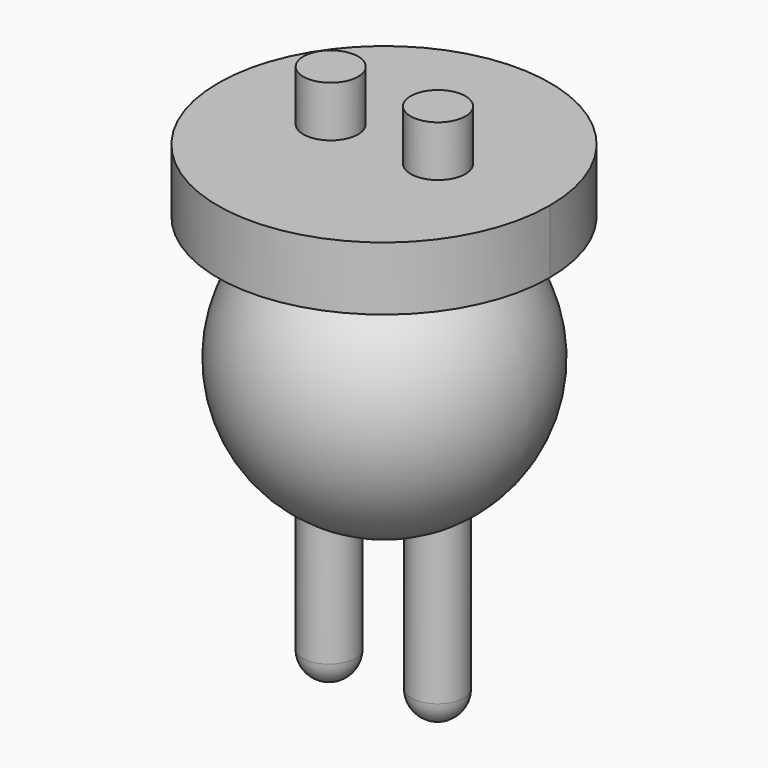
from build123d import *

# Parameters (mm, degrees)
F0_R     = 10.7853529021
F7_DEPTH = 45
F0_R_2   = 65.2735484533
F8_DEPTH = 25


with BuildPart() as f2:
    # F1 (on Front) → F2 (revolve)
    with BuildSketch(Plane.XZ):
        with BuildLine():
            ThreePointArc((0, -105.0551608205), (39.6174808002, -88.645062966), (56.0275786547, -49.0275821658))
            ThreePointArc((56.0275786547, -49.0275821658), (39.6174808002, -9.4101013656), (0, 6.9999964889))
            Line((0, 6.9999964889), (0, -105.0551608205))
        make_face()
    revolve(axis=Axis((0, 0, -49.0275821658), (0, 0, -1)))

    # F3 (on Front) → F4 (revolve)
    with BuildSketch(Plane.XZ):
        with BuildLine():
            Line((-21.801807452, -156.9885462523), (-32.1567505598, -156.9885462523))
            ThreePointArc((-32.1567505598, -156.9885462523), (-29.1238579423, -164.3105967426), (-21.801807452, -167.3434893601))
            Line((-21.801807452, -167.3434893601), (-21.801807452, -156.9885462523))
        make_face()
        with BuildLine():
            Line((-32.1567505598, -87.396197021), (-32.1567505598, -156.9885462523))
            ThreePointArc((-32.1567505598, -156.9885462523), (-29.1238579423, -149.6664957619), (-21.801807452, -146.6336031444))
            Line((-21.801807452, -146.6336031444), (-21.801807452, -87.396197021))
            Line((-21.801807452, -87.396197021), (-32.1567505598, -87.396197021))
        make_face()
        with BuildLine():
            ThreePointArc((-21.801807452, -146.6336031444), (-29.1238579423, -149.6664957619), (-32.1567505598, -156.9885462523))
            Line((-32.1567505598, -156.9885462523), (-21.801807452, -156.9885462523))
            Line((-21.801807452, -156.9885462523), (-21.801807452, -146.6336031444))
        make_face()
    revolve(axis=Axis((-21.801807452, 0, -127.3698431905), (0, 0, 1)))

    # F5 (on Front) → F6 (revolve)
    with BuildSketch(Plane.XZ):
        with BuildLine():
            Line((20.9296178073, -146.5023671743), (20.9296178073, -167.2122533899))
            ThreePointArc((20.9296178073, -167.2122533899), (28.2516682976, -164.1793607724), (31.2845609151, -156.8573102821))
            ThreePointArc((31.2845609151, -156.8573102821), (28.2516682976, -149.5352597917), (20.9296178073, -146.5023671743))
        make_face()
        with BuildLine():
            Line((20.9296178073, -87.2649610508), (20.9296178073, -146.5023671743))
            ThreePointArc((20.9296178073, -146.5023671743), (28.2516682976, -149.5352597917), (31.2845609151, -156.8573102821))
            Line((31.2845609151, -156.8573102821), (31.2845609151, -87.2649610508))
            Line((31.2845609151, -87.2649610508), (20.9296178073, -87.2649610508))
        make_face()
    revolve(axis=Axis((20.9296178073, 0, -127.2386072204), (0, 0, 1)))

    # F0 (on Top) → F7 (join)
    with BuildSketch(Plane.XY):
        with Locations((21.1290447041, 0)):
            Circle(F0_R)
        with Locations((-21.1290447041, 0)):
            Circle(F0_R)
    extrude(amount=F7_DEPTH)

    # F0 (on Top) → F8 (join)
    with BuildSketch(Plane.XY):
        Circle(F0_R_2)
        with Locations((-21.1290447041, 0)):
            Circle(F0_R, mode=Mode.SUBTRACT)
        with Locations((21.1290447041, 0)):
            Circle(F0_R, mode=Mode.SUBTRACT)
        with Locations((0, -0.3733891062)):
            Circle(F0_R_2)
    extrude(amount=F8_DEPTH)


solid = f2.part
